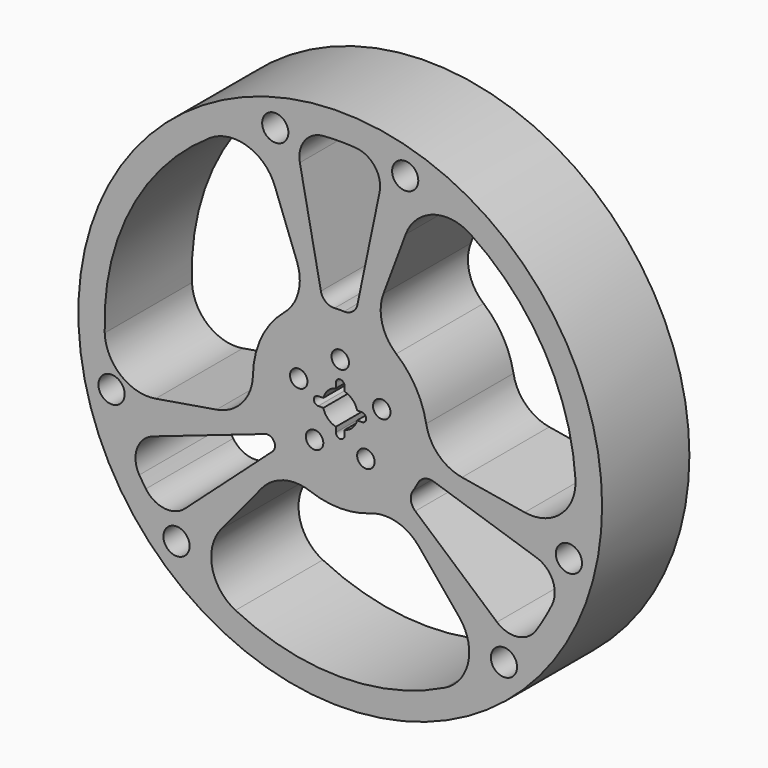
from build123d import *

# Parameters (mm, degrees)
F0_R     = 60
F0_R_2   = 3
F0_R_3   = 15
F0_R_4   = 2
F1_DEPTH = 25


# Not quite as in the source:
# - a feature names something its author has since deleted; it is built from what else it names


with BuildPart() as f1:
    # F0 (on Front) → F1 (new body)
    with BuildSketch(Plane.XZ):
        Circle(F0_R)
        with Locations((-37.5115520048, -38.8443492183)):
            Circle(F0_R_2, mode=Mode.SUBTRACT)
        with BuildLine():
            ThreePointArc((-17.9991214641, -21.8181490168), (-12.909542723, -18.5322896083), (-6.8568272685, -18.7878662921))
            ThreePointArc((-6.8568272685, -18.7878662921), (0.003827401, -19.9999996338), (6.864017636, -18.7852405333))
            ThreePointArc((6.864017636, -18.7852405333), (12.9220689894, -18.5288245474), (18.0146364939, -21.8199476948))
            Line((18.0146364939, -21.8199476948), (27.2720618955, -33.0586128775))
            ThreePointArc((27.2720618955, -33.0586128775), (29.3324432338, -41.5072979988), (23.9974181864, -48.3748273422))
            ThreePointArc((23.9974181864, -48.3748273422), (0, -54), (-23.9974181864, -48.3748273422))
            ThreePointArc((-23.9974181864, -48.3748273422), (-29.3332198415, -41.5036623321), (-27.2673324169, -33.0528755612))
            Line((-27.2673324169, -33.0528755612), (-17.9991214641, -21.8181490168))
        make_face(mode=Mode.SUBTRACT)
        with BuildLine():
            ThreePointArc((-44.5250909536, -30.5534985815), (-45.2912230512, -29.4058687089), (-46.0277820813, -28.2390381684))
            ThreePointArc((-46.0277820813, -28.2390381684), (-46.5604522686, -23.0733436974), (-42.8629692739, -19.4268719232))
            Line((-42.8629692739, -19.4268719232), (-16.9967316552, -10.5409256254))
            ThreePointArc((-16.9967316552, -10.5409256254), (-15.120110809, -11.5154453431), (-15.5299138764, -13.5899226089))
            Line((-15.5299138764, -13.5899226089), (-16.9726013847, -14.8870728677))
            Line((-16.9726013847, -14.8870728677), (-17.1078816805, -15.0240893401))
            Line((-17.1078816805, -15.0240893401), (-35.5662381193, -31.6203804252))
            ThreePointArc((-35.5662381193, -31.6203804252), (-40.2873666152, -33.116567588), (-44.5250909536, -30.5534985815))
        make_face(mode=Mode.SUBTRACT)
        with Locations((-52.3959692189, -13.0637823624)):
            Circle(F0_R_2, mode=Mode.SUBTRACT)
        with Locations((37.5115520048, -38.8443492183)):
            Circle(F0_R_2, mode=Mode.SUBTRACT)
        with BuildLine():
            Line((21.3985322272, -7.6356383993), (45.0061435827, -15.3247300238))
            ThreePointArc((45.0061435827, -15.3247300238), (48.6715278542, -18.6865524369), (48.5414946952, -23.6584719025))
            ThreePointArc((48.5414946952, -23.6584719025), (46.8021183332, -26.9362528857), (44.8417435514, -30.0868415635))
            ThreePointArc((44.8417435514, -30.0868415635), (40.6476491874, -32.6918461445), (35.9197630861, -31.2693239428))
            Line((35.9197630861, -31.2693239428), (17.1994124126, -14.9726488191))
            ThreePointArc((17.1994124126, -14.9726488191), (16.1962922773, -13.1122239789), (16.6688649306, -11.0521012448))
            ThreePointArc((16.6688649306, -11.0521012448), (17.2612476069, -10.1019468943), (17.7995287636, -9.1201302509))
            ThreePointArc((17.7995287636, -9.1201302509), (19.3255292381, -7.7148076154), (21.3985322272, -7.6356383993))
        make_face(mode=Mode.SUBTRACT)
        with Locations((52.3959692189, -13.0637823624)):
            Circle(F0_R_2, mode=Mode.SUBTRACT)
        with BuildLine():
            Line((-14.9909636957, 40.1406403471), (-9.8955105801, 26.4967709421))
            ThreePointArc((-9.8955105801, 26.4967709421), (-9.5946622296, 20.4461367535), (-12.8423558576, 15.3321197499))
            ThreePointArc((-12.8423558576, 15.3321197499), (-18.0436420311, 8.6271074095), (-19.9965959104, 0.3689877998))
            ThreePointArc((-19.9965959104, 0.3689877998), (-22.4237136521, -5.9792994979), (-28.3480846215, -9.3099872294))
            Line((-28.3480846215, -9.3099872294), (-42.3172195747, -11.6422803342))
            ThreePointArc((-42.3172195747, -11.6422803342), (-50.2710809676, -9.5390364788), (-53.9558535504, -2.1830867246))
            ThreePointArc((-53.9558535504, -2.1830867246), (-48.0998424018, 24.5439434672), (-29.8951202889, 44.9697874457))
            ThreePointArc((-29.8951202889, 44.9697874457), (-21.276616009, 46.1551447236), (-14.9909636957, 40.1406403471))
        make_face(mode=Mode.SUBTRACT)
        with BuildLine():
            Line((-4.4279652677, 22.3694685585), (-9.2474940163, 46.7170617057))
            ThreePointArc((-9.2474940163, 46.7170617057), (-8.1285920064, 51.5258593406), (-3.7819096653, 53.8674034949))
            ThreePointArc((-3.7819096653, 53.8674034949), (-0.1220878193, 53.9998619865), (3.5382955571, 53.8839536834))
            ThreePointArc((3.5382955571, 53.8839536834), (7.9230697986, 51.5261035304), (9.0182868498, 46.6695407434))
            Line((9.0182868498, 46.6695407434), (3.9392668723, 22.3644794699))
            ThreePointArc((3.9392668723, 22.3644794699), (2.8434498256, 20.6092434876), (0.8719123918, 19.9809851804))
            ThreePointArc((0.8719123918, 19.9809851804), (-0.2100325239, 19.9988971281), (-1.2913626084, 19.9582660222))
            ThreePointArc((-1.2913626084, 19.9582660222), (-3.31345185, 20.5735591973), (-4.4279652677, 22.3694685585))
        make_face(mode=Mode.SUBTRACT)
        with Locations((-14.8844172141, 51.9081315807)):
            Circle(F0_R_2, mode=Mode.SUBTRACT)
        Circle(F0_R_3, mode=Mode.SUBTRACT)
        with BuildLine():
            ThreePointArc((12.8423558576, 15.3321197499), (9.5946622296, 20.4461367535), (9.8955105801, 26.4967709421))
            Line((9.8955105801, 26.4967709421), (14.9909636957, 40.1406403471))
            ThreePointArc((14.9909636957, 40.1406403471), (21.276616009, 46.1551447236), (29.8951202889, 44.9697874457))
            ThreePointArc((29.8951202889, 44.9697874457), (46.7619600734, 27.0059084294), (53.8916763243, 3.4186580637))
            ThreePointArc((53.8916763243, 3.4186580637), (50.6128315094, -4.6370491105), (42.2649270201, -7.0778956919))
            Line((42.2649270201, -7.0778956919), (27.9019654451, -4.6798491157))
            ThreePointArc((27.9019654451, -4.6798491157), (22.506844055, -1.9164656047), (19.6991831261, 3.4557465422))
            ThreePointArc((19.6991831261, 3.4557465422), (17.3205080757, 10), (12.8423558576, 15.3321197499))
        make_face(mode=Mode.SUBTRACT)
        with Locations((14.8844172141, 51.9081315807)):
            Circle(F0_R_2, mode=Mode.SUBTRACT)
        Circle(F0_R_3)
        with Locations((-5.8778525229, -8.0901699437)):
            Circle(F0_R_4, mode=Mode.SUBTRACT)
        with BuildLine():
            ThreePointArc((-3.8729833462, 1), (-2.8284271247, 2.8284271247), (-1, 3.8729833462))
            Line((-1, 3.8729833462), (-1, 5))
            ThreePointArc((-1, 5), (0, 6), (1, 5))
            Line((1, 5), (1, 3.8729833462))
            ThreePointArc((1, 3.8729833462), (2.8284271247, 2.8284271247), (3.8729833462, 1))
            Line((3.8729833462, 1), (4.9514505081, 1))
            ThreePointArc((4.9514505081, 1), (5.9514505081, 0), (4.9514505081, -1))
            Line((4.9514505081, -1), (3.8729833462, -1))
            ThreePointArc((3.8729833462, -1), (2.8284271247, -2.8284271247), (1, -3.8729833462))
            Line((1, -3.8729833462), (1, -5.0126444548))
            ThreePointArc((1, -5.0126444548), (0, -6.0126444548), (-1, -5.0126444548))
            Line((-1, -5.0126444548), (-1, -3.8729833462))
            ThreePointArc((-1, -3.8729833462), (-2.8284271247, -2.8284271247), (-3.8729833462, -1))
            Line((-3.8729833462, -1), (-5.0453338772, -1))
            ThreePointArc((-5.0453338772, -1), (-6.0453338772, 0), (-5.0453338772, 1))
            Line((-5.0453338772, 1), (-3.8729833462, 1))
        make_face(mode=Mode.SUBTRACT)
        with Locations((5.8778525229, -8.0901699437)):
            Circle(F0_R_4, mode=Mode.SUBTRACT)
        with Locations((-9.510565163, 3.0901699437)):
            Circle(F0_R_4, mode=Mode.SUBTRACT)
        with Locations((9.510565163, 3.0901699437)):
            Circle(F0_R_4, mode=Mode.SUBTRACT)
        with Locations((0, 10)):
            Circle(F0_R_4, mode=Mode.SUBTRACT)
    extrude(amount=F1_DEPTH)


solid = f1.part
